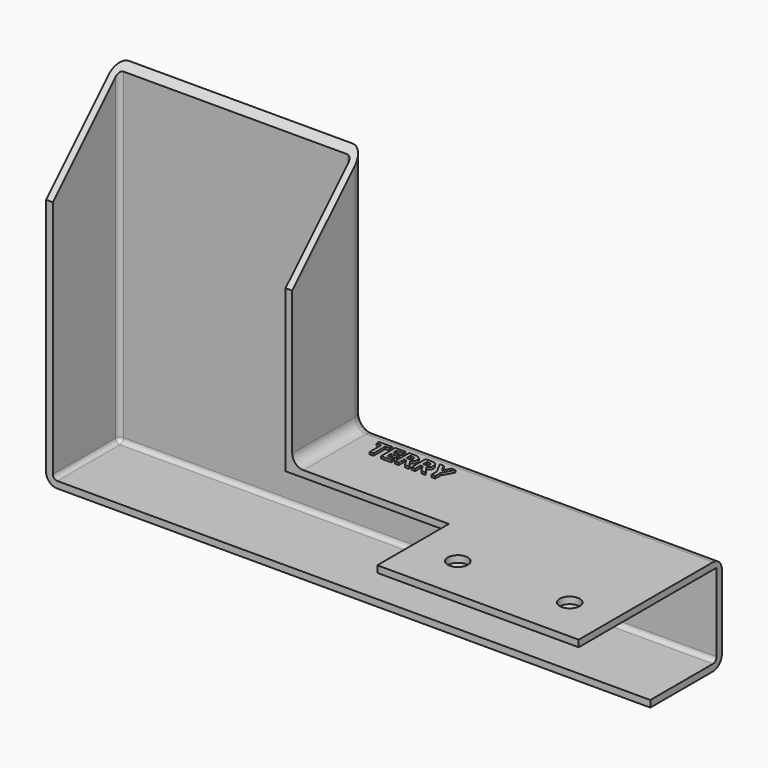
from build123d import *

# Parameters (mm, degrees)
F1_DEPTH      = 1.5
F3_DEPTH      = 18.5
F4_W          = 45
F4_H          = 1.5
F5_DEPTH      = 20
F6_R          = 2.25
F7_DEPTH      = 1.5
F9_DEPTH      = 55
F10_R         = 1
F11_R         = 2.5
F12_TEXT_SIZE = 5.5555555556
F13_DEPTH     = 0.5


# Not quite as in the source:
# - Text() gives the source's letters only with a copy of the font that has no kerning and outlines rounded to 1/6400 em; it was checked with that copy


with BuildPart() as f1:
    # F0 (on Front) → F1 (new body)
    with BuildSketch(Plane.XZ):
        Polygon((80, 0), (0, 0), (0, 54.5), (-55, 54.5), (-55, -21.5), (80, -21.5), align=None)
    extrude(amount=F1_DEPTH)

    # F2 (on face) → F3 (join)
    with BuildSketch(Plane.XZ.offset(1.5)):
        Polygon((-53.5, 54.5), (-55, 54.5), (-55, -21.5), (80, -21.5), (80, -20), (-53.5, -20), align=None)
        Polygon((0, 54.5), (-1.5, 54.5), (-1.5, -1.5), (80, -1.5), (80, 0), (0, 0), align=None)
    extrude(amount=F3_DEPTH)

    # F4 (on face) → F5 (join)
    with BuildSketch(Plane.XZ.offset(20)):
        with Locations((57.5, -0.75)):
            Rectangle(F4_W, F4_H)
    extrude(amount=F5_DEPTH)

    # F6 (on face) → F7 (cut, through all)
    with BuildSketch(Plane.XY):
        with Locations((45, -30)):
            Circle(F6_R)
        with Locations((70, -30)):
            Circle(F6_R)
    extrude(amount=-F7_DEPTH, mode=Mode.SUBTRACT)

    # F8 (on face) → F9 (cut)
    with BuildSketch(Plane(origin=(-55, 0, 0), x_dir=(0, -1, 0), z_dir=(-1, 0, 0))):
        Polygon((0, 54.5), (20, 34.5), (20, 54.5), align=None)
    extrude(amount=-F9_DEPTH, mode=Mode.SUBTRACT)

    # F10
    f10_edges = [f1.edges().sort_by_distance(p)[0] for p in [
        (-1.5, -1.5, 25.75),
        (13.25, -1.5, -20),
        (-53.5, -1.5, 16.5),
        (-53.5, -10.75, -20),
    ]]
    fillet(f10_edges, radius=F10_R)

    # F11
    f11_edges = [f1.edges().sort_by_distance(p)[0] for p in [
        (12.5, 0, -21.5),
        (40, 0, 0),
        (0, 0, 27.25),
        (-55, 0, 16.5),
        (-55, -10, -21.5),
        (0, -10, 0),
    ]]
    fillet(f11_edges, radius=F11_R)

    # F12 (on face) → F13 (join)
    with BuildSketch(Plane.XY):
        with Locations((6.625, -8.125)):
            Text('TERRY', F12_TEXT_SIZE, font='Open Sans', font_style=FontStyle.BOLD, text_align=(TextAlign.LEFT, TextAlign.BOTTOM))
    extrude(amount=F13_DEPTH)


solid = f1.part
